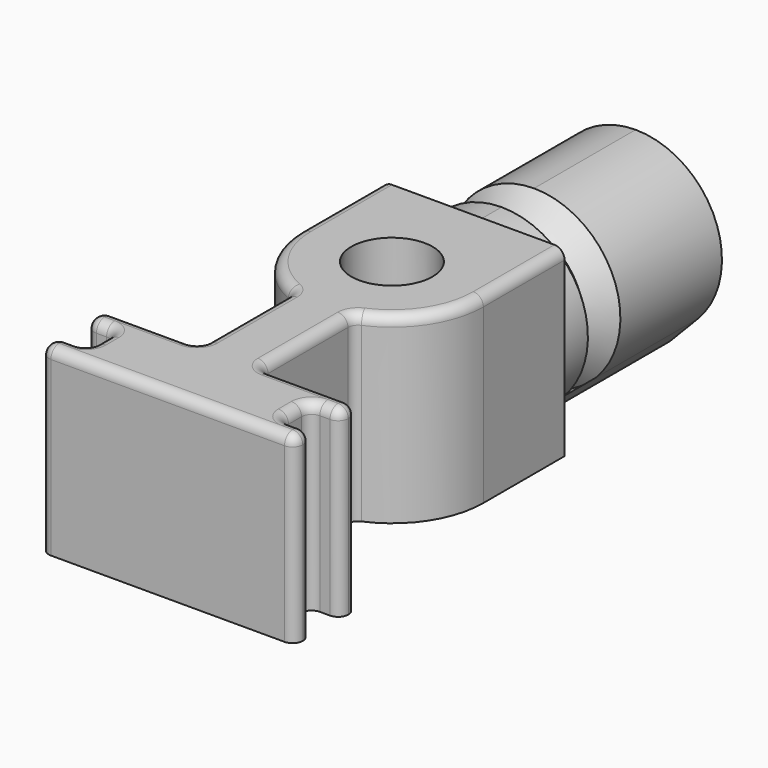
from build123d import *

# Parameters (mm, degrees)
F0_R      = 4
F1_DEPTH  = 18
F3_R      = 0.99999
F6_DEPTH  = 20
F8_DEPTH  = 30
F9_SIZE   = 1
F10_R     = 5
F11_DEPTH = 3.5


# Not quite as in the source:
# - two fillets or chamfers of one size are made in one step
# - a fillet or chamfer is up to 0.001 mm smaller than in the source, because OpenCascade refuses the exact size


with BuildPart() as f1:
    # F0 (on Top) → F1 (new body)
    with BuildSketch(Plane.XY):
        with BuildLine():
            Line((3, -20), (3, -8.4852813742))
            ThreePointArc((3, -8.4852813742), (7.3484692283, -5.1961524227), (9, 0))
            Line((9, 0), (9, 30))
            Line((9, 30), (-9, 30))
            Line((-9, 30), (-9, 0))
            ThreePointArc((-9, 0), (-7.3484692283, -5.1961524227), (-3, -8.4852813742))
            Line((-3, -8.4852813742), (-3, -20))
            Line((-3, -20), (-12.5, -20))
            Line((-12.5, -20), (-12.5, -22))
            Line((-12.5, -22), (-9.5, -22))
            Line((-9.5, -22), (-9.5, -25.6))
            Line((-9.5, -25.6), (-12.5, -25.6))
            Line((-12.5, -25.6), (-12.5, -27.6))
            Line((-12.5, -27.6), (0, -27.6))
            Line((0, -27.6), (12.5, -27.6))
            Line((12.5, -27.6), (12.5, -25.6))
            Line((12.5, -25.6), (9.5, -25.6))
            Line((9.5, -25.6), (9.5, -22))
            Line((9.5, -22), (12.5, -22))
            Line((12.5, -22), (12.5, -20))
            Line((12.5, -20), (3, -20))
        make_face()
        Circle(F0_R, mode=Mode.SUBTRACT)
    extrude(amount=F1_DEPTH)

    # F3 (radius 1 in the source; OpenCascade refuses exactly that, so slightly less here)
    f3_edges = [f1.edges().sort_by_distance(p)[0] for p in [
        (3, -20, 9),
        (-3, -20, 9),
        (3, -8.485281, 9),
        (12.5, -27.6, 9),
        (-12.5, -27.6, 9),
        (-9.5, -25.6, 9),
        (-12.5, -25.6, 9),
        (-9.5, -22, 9),
        (-12.5, -22, 9),
        (-12.5, -20, 9),
        (12.5, -25.6, 9),
        (9.5, -25.6, 9),
        (9.5, -22, 9),
        (12.5, -22, 9),
        (12.5, -20, 9),
        (3, -14.242641, 18),
        (7.348469, -5.196152, 18),
        (9, 15, 18),
        (-9, 15, 18),
        (-7.348469, -5.196152, 18),
        (-3, -14.242641, 18),
        (-7.75, -20, 18),
        (-12.5, -21, 18),
        (-11, -22, 18),
        (-9.5, -23.8, 18),
        (-11, -25.6, 18),
        (-12.5, -26.6, 18),
        (0, -27.6, 18),
        (12.5, -26.6, 18),
        (11, -25.6, 18),
        (9.5, -23.8, 18),
        (11, -22, 18),
        (12.5, -21, 18),
        (7.75, -20, 18),
        (-3, -8.485281, 9),
    ]]
    fillet(f3_edges, radius=F3_R)

    # F5 (on face) → F6 (cut)
    with BuildSketch(Plane(origin=(0, 30, 0), x_dir=(-1, 0, 0), z_dir=(0, 1, 0))):
        with BuildLine():
            Line((-11.1393053085, 0), (-9, 0))
            Line((-9, 0), (-9, 17.00001))
            ThreePointArc((-9, 17.00001), (-8.7071097101, 17.7071097101), (-8.00001, 18))
            Line((-8.00001, 18), (8.00001, 18))
            ThreePointArc((8.00001, 18), (8.7071097101, 17.7071097101), (9, 17.00001))
            Line((9, 17.00001), (9, 21.8532588333))
            Line((9, 21.8532588333), (-11.1393053085, 21.8532588333))
            Line((-11.1393053085, 21.8532588333), (-11.1393053085, 0))
        make_face()
        with BuildLine():
            Line((6.1143883029, 2.836985475), (3.3747432753, 0))
            Line((3.3747432753, 0), (9, 0))
            Line((9, 0), (9, 17.00001))
            ThreePointArc((9, 17.00001), (8.7071097101, 17.7071097101), (8.00001, 18))
            Line((8.00001, 18), (-8.00001, 18))
            ThreePointArc((-8.00001, 18), (-8.7071097101, 17.7071097101), (-9, 17.00001))
            Line((-9, 17.00001), (-9, 0))
            Line((-9, 0), (-3.3747432753, 0))
            Line((-3.3747432753, 0), (-6.1143883029, 2.836985475))
            ThreePointArc((-6.1143883029, 2.836985475), (-7.8242912543, 12.0627962161), (0, 17.2415816239))
            ThreePointArc((0, 17.2415816239), (7.8242912543, 12.0627962161), (6.1143883029, 2.836985475))
        make_face()
    extrude(amount=-F6_DEPTH, mode=Mode.SUBTRACT)

    # F7 (on face) → F8 (cut)
    with BuildSketch(Plane(origin=(0, 30, 0), x_dir=(-1, 0, 0), z_dir=(0, 1, 0))):
        Polygon((4.5, 8.7415816239), (0, 14.1044727906), (-4.5, 8.7415816239), (0, 3.3786904573), align=None)
    extrude(amount=-F8_DEPTH, mode=Mode.SUBTRACT)

    # F9
    f9_edges = [f1.edges().sort_by_distance(p)[0] for p in [
        (0, 17, 3.37869),
    ]]
    chamfer(f9_edges, length=F9_SIZE)

    # F10 (on face) → F11 (join)
    with BuildSketch(Plane(origin=(0, 0, 0), x_dir=(1, 0, 0), z_dir=(0, 0, -1))):
        Circle(F10_R)
    extrude(amount=-F11_DEPTH)

    # F12 (on Right) → F13 (revolve, cut)
    with BuildSketch(Plane.YZ):
        Polygon((17.5, 17.2415816239), (13.5, 17.2415816239), (15.5, 15.2415816239), align=None)
    revolve(axis=Axis((0, 30, 8.7415816239), (0, 1, 0)), mode=Mode.SUBTRACT)


solid = f1.part
